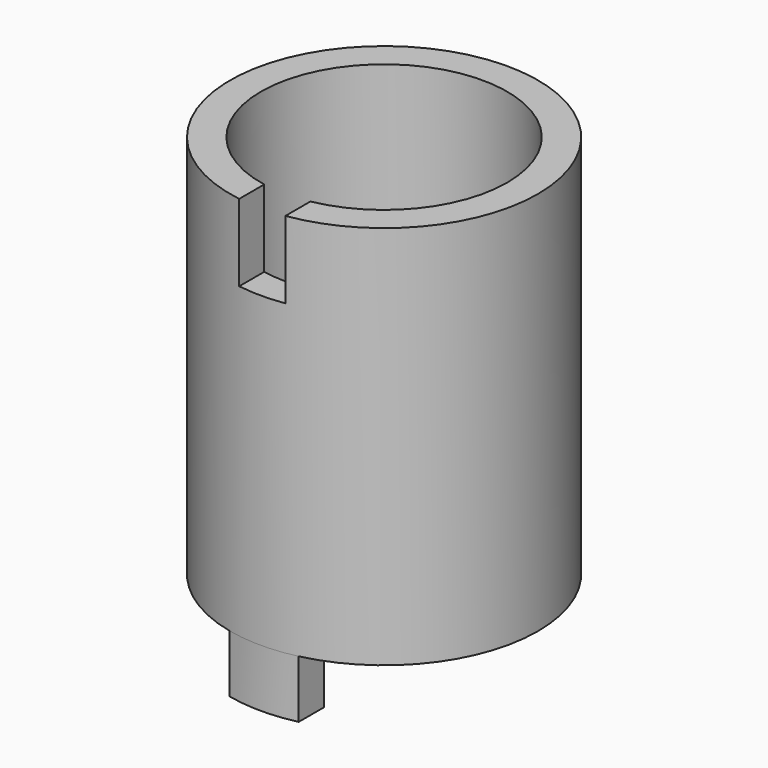
from build123d import *

# Parameters (mm, degrees)
F0_R          = 5.08
F0_R_2        = 4.064
F1_DEPTH      = 12.7
F2_W          = 1.524
F2_H          = 2.54
F3_DEPTH      = 25.4
F5_END_RADIUS = 5.08
F4_W          = 2.286
F4_H          = 1.905
F5_REACH      = 8.0567051265
F6_END_RADIUS = 4.064
F6_REACH      = 8.0567051265


with BuildPart() as f1:
    # F0 (on Top) → F1 (new body)
    with BuildSketch(Plane.XY):
        Circle(F0_R)
        Circle(F0_R_2, mode=Mode.SUBTRACT)
    extrude(amount=F1_DEPTH)

    # F2 (on Front) → F3 (cut)
    with BuildSketch(Plane.XZ):
        with Locations((0, 11.43)):
            Rectangle(F2_W, F2_H)
    extrude(amount=F3_DEPTH, mode=Mode.SUBTRACT)

    f5_end = (Plane(origin=(0, 0, 6.35), x_dir=(-1, 0, 0), z_dir=(0, 0, -1)) * Cylinder(F5_END_RADIUS, 54.4665691842, mode=Mode.PRIVATE)).faces().sort_by_distance((-5.08, 0, 6.35))[0]
    # F4 (on Front) → F5 (join, up to the whole of a round face its end follows)
    with BuildSketch(Plane.XZ):
        with Locations((0, -0.9525)):
            Rectangle(F4_W, F4_H)
    f5_long = extrude(amount=F5_REACH, mode=Mode.PRIVATE)
    add(split(f5_long, bisect_by=f5_end, keep=Keep.BOTTOM, mode=Mode.PRIVATE))

    f6_end = (Plane(origin=(0, 0, 6.35), x_dir=(-1, 0, 0), z_dir=(0, 0, -1)) * Cylinder(F6_END_RADIUS, 57.0893653975, mode=Mode.PRIVATE)).faces().sort_by_distance((-4.064, 0, 6.35))[0]
    # F4 (on Front) → F6 (cut, up to the whole of a round face its end follows)
    with BuildSketch(Plane.XZ):
        with Locations((0, -0.9525)):
            Rectangle(F4_W, F4_H)
    f6_long = extrude(amount=F6_REACH, mode=Mode.PRIVATE)
    add(split(f6_long, bisect_by=f6_end, keep=Keep.BOTTOM, mode=Mode.PRIVATE), mode=Mode.SUBTRACT)


solid = f1.part
